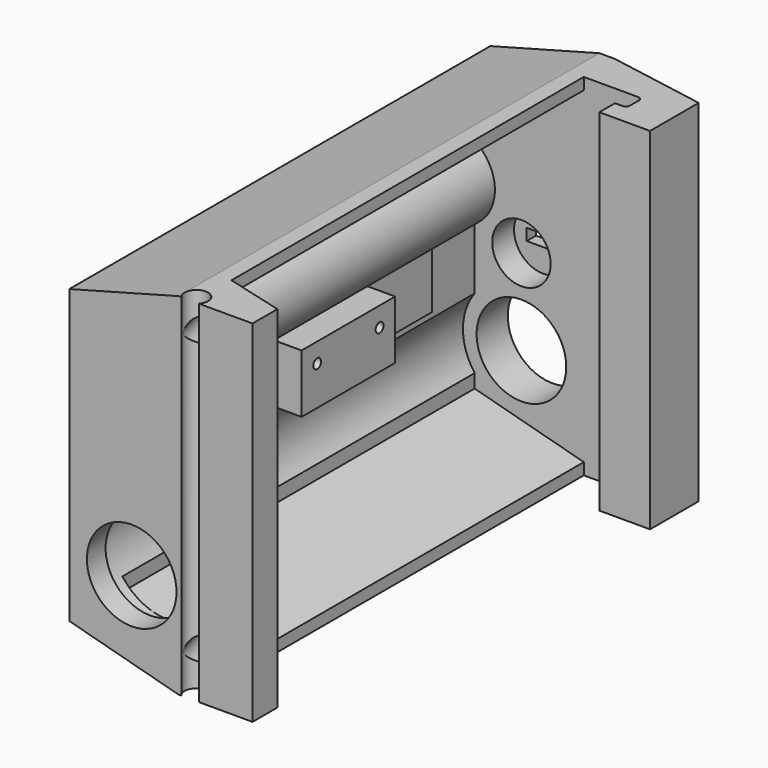
from build123d import *

# Parameters (mm, degrees)
F1_DEPTH  = 45
F2_SIZE2  = 7.502567
F2_SIZE   = 27.99999
F3_SIZE2  = 7.502567
F3_SIZE   = 27.99999
F5_DEPTH  = 113
F6_R      = 11.5
F7_DEPTH  = 135.001
F8_R      = 15
F9_DEPTH  = 6
F10_DEPTH = 113
F11_W     = 30
F11_H     = 15
F12_DEPTH = 22
F13_R     = 1.25
F14_DEPTH = 15
F15_W     = 8.5
F15_H     = 3
F16_DEPTH = 10
F17_R     = 7.5
F18_DEPTH = 7
F19_W     = 25
F19_H     = 15
F20_DEPTH = 5
F21_SIZE2 = 4.4081745177
F21_SIZE  = 25
F25_R     = 11
F26_DEPTH = 92
F27_R     = 1


# Not quite as in the source:
# - a fillet or chamfer is up to 0.001 mm smaller than in the source, because OpenCascade refuses the exact size
# - a pattern or mirror of a feature is missing from the dataset's text; its kind, count and spacing are read off the source's solid


with BuildPart() as f1:
    # F0 (on Top) → F1 (new body, symmetric)
    with BuildSketch(Plane.XY):
        with BuildLine():
            Line((0, -113), (0, 0))
            Line((0, 0), (15, 0))
            Line((15, 0), (15, -5))
            Line((15, -5), (12, -5))
            Line((12, -5), (12, -10))
            Line((12, -10), (25, -10))
            Line((25, -10), (25, 10))
            Line((25, 10), (-32, 10))
            Line((-32, 10), (-32, -125))
            Line((-32, -125), (-3.2360679775, -125))
            ThreePointArc((-3.2360679775, -125), (-1, -120), (1.2360679775, -125))
            Line((1.2360679775, -125), (15, -125))
            Line((15, -125), (15, -117.0192378865))
            Line((15, -117.0192378865), (0, -113))
        make_face()
    extrude(amount=F1_DEPTH, both=True)

    # F2 (size 28 and 7.5025773881 in the source; OpenCascade refuses exactly that, so slightly less here)
    f2_edges = [f1.edges().sort_by_distance(p)[0] for p in [
        (-32, -57.5, 45),
    ]]
    f2_side = f1.faces().sort_by_distance((-13.040115, -54.60791, 45))[0]
    chamfer(f2_edges, length=F2_SIZE, length2=F2_SIZE2, reference=f2_side)

    # F3 (size 28 and 7.5025773881 in the source; OpenCascade refuses exactly that, so slightly less here)
    f3_edges = [f1.edges().sort_by_distance(p)[0] for p in [
        (-32, -57.5, -45),
    ]]
    f3_side = f1.faces().sort_by_distance((-13.040115, -54.60791, -45))[0]
    chamfer(f3_edges, length=F3_SIZE, length2=F3_SIZE2, reference=f3_side)

    # F4 (on face) → F5 (cut)
    with BuildSketch(Plane.XZ):
        Polygon((0, -42), (0, 0), (0, 42), (-28, 34.4974226119), (-28, 0), (-28, -34.4974226119), align=None)
    extrude(amount=F5_DEPTH, mode=Mode.SUBTRACT)

    # F6 (on face) → F7 (cut, through all)
    with BuildSketch(Plane.XZ.offset(125)):
        with Locations((-16, -22)):
            Circle(F6_R)
    extrude(amount=-F7_DEPTH, mode=Mode.SUBTRACT)

    # F8 (on face) → F9 (cut)
    with BuildSketch(Plane(origin=(0, -113, 0), x_dir=(-1, 0, 0), z_dir=(0, 1, 0))):
        with Locations((16, -22)):
            Circle(F8_R)
    extrude(amount=-F9_DEPTH, mode=Mode.SUBTRACT)

    # F8 (on face) → F10 (cut, through all)
    with BuildSketch(Plane(origin=(0, -113, 0), x_dir=(-1, 0, 0), z_dir=(0, 1, 0))):
        with Locations((16, -22)):
            Circle(F8_R)
    extrude(amount=F10_DEPTH, mode=Mode.SUBTRACT)

    # F11 (on face) → F12 (join)
    with BuildSketch(Plane.YZ.offset(-28)):
        with Locations((-68, 7.5)):
            Rectangle(F11_W, F11_H)
    extrude(amount=F12_DEPTH)

    # F13 (on face) → F14 (cut)
    with BuildSketch(Plane.YZ.offset(-6)):
        with Locations((-78, 10)):
            Circle(F13_R)
        with Locations((-58, 10)):
            Circle(F13_R)
    extrude(amount=-F14_DEPTH, mode=Mode.SUBTRACT)

    # F15 (on face) → F16 (cut, through all)
    with BuildSketch(Plane(origin=(0, 10, 0), x_dir=(-1, 0, 0), z_dir=(0, 1, 0))):
        with Locations((16, 0)):
            Rectangle(F15_W, F15_H)
    extrude(amount=-F16_DEPTH, mode=Mode.SUBTRACT)

    # F17 (on face) → F18 (cut)
    with BuildSketch(Plane.XZ):
        with Locations((-16, 0)):
            Circle(F17_R)
    extrude(amount=-F18_DEPTH, mode=Mode.SUBTRACT)

    # F19 (on face) → F20 (join)
    with BuildSketch(Plane.YZ.offset(-28)):
        with Locations((-100.5, 0)):
            Rectangle(F19_W, F19_H)
        with Locations((-32.5, 0)):
            Rectangle(F19_W, F19_H)
    extrude(amount=F20_DEPTH)

    # F21
    f21_edges = [f1.edges().sort_by_distance(p)[0] for p in [
        (25, 10, 0),
    ]]
    f21_side = f1.faces().sort_by_distance((-1.370356, 10, 2.040759))[0]
    chamfer(f21_edges, length=F21_SIZE, length2=F21_SIZE2, reference=f21_side)

    # F23 (on offset) → F24 (revolve, cut)
    with BuildSketch(Plane.XY.offset(36)):
        Polygon((-4.9269355532, -99.7771988864), (-7.7971363015, -100.6500950226), (-1, -123), (1.8702007483, -122.1271038638), align=None)
    f24 = revolve(axis=Axis((-4.3985681508, -111.8250475113, 36), (0.2909653787, -0.9567335828, 0)), mode=Mode.SUBTRACT)

    # F24_copies: F24 across plane
    add(f24.mirror(Plane(origin=(0, 0, -1.1e-05), x_dir=(-1, 0, 0), z_dir=(0, 0, -1))), mode=Mode.SUBTRACT)

    # F27
    f27_edges = [f1.edges().sort_by_distance(p)[0] for p in [
        (15, 0, 0),
        (15, -5, 0),
    ]]
    fillet(f27_edges, radius=F27_R)


with BuildPart() as f26:
    # F25 (on face) → F26 (new body)
    with BuildSketch(Plane(origin=(0, -113, 0), x_dir=(-1, 0, 0), z_dir=(0, 1, 0))):
        with Locations((17, 26.0568257442)):
            Circle(F25_R)
    extrude(amount=F26_DEPTH)


solid = Compound([f1.part, f26.part])
